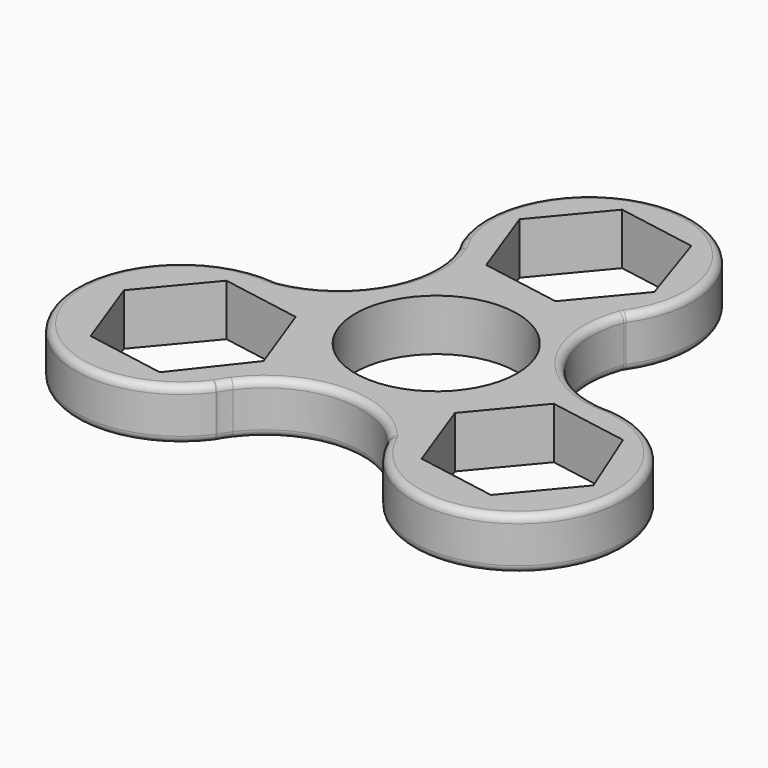
from build123d import *

# Parameters (mm, degrees)
F0_R     = 11
F1_DEPTH = 7
F2_F1_R  = 1
F2_F2_R  = 1
F2_F3_R  = 0.9999


# Not quite as in the source:
# - a fillet or chamfer is up to 0.001 mm smaller than in the source, because OpenCascade refuses the exact size


with BuildPart() as f1:
    # F0 (on Top) → F1 (new body)
    with BuildSketch(Plane.XY):
        with BuildLine():
            ThreePointArc((22.2086241305, 0.0798641866), (12.5198905979, 6.2741646263), (11.4517572715, 17.7240557437))
            ThreePointArc((11.4517572715, 17.7240557437), (1.6771991192, 39.973348249), (-13.0734749912, 20.6603832424))
            ThreePointArc((-13.0734749912, 20.6603832424), (-12.5180191421, 19.6665029377), (-12.0509754633, 18.6281390985))
            ThreePointArc((-12.0509754633, 18.6281390985), (-12.8422160416, 7.2882657582), (-22.2022373142, 0.8377781175))
            ThreePointArc((-22.2022373142, 0.8377781175), (-37.1071375636, -19.0809555006), (-12.384246779, -21.854161524))
            ThreePointArc((-12.384246779, -21.854161524), (-11.9079611923, -21.041379868), (-11.3744869733, -20.2649346104))
            ThreePointArc((-11.3744869733, -20.2649346104), (-1.1159335609, -14.9703009767), (9.3470139898, -19.8485990384))
            ThreePointArc((9.3470139898, -19.8485990384), (34.0495934391, -22.7972544861), (24.0898149129, 0))
            ThreePointArc((24.0898149129, 0), (23.1477825578, 0.0060845895), (22.2086241305, 0.0798641866))
        make_face()
        Polygon((-11.7877372927, -14.5967135669), (-18.7727350589, -23.4860221006), (-29.7069392796, -21.574693228), (-33.5187820314, -11.1497301664), (-26.3964205624, -2.6360959774), (-15.4622163417, -4.5474248499), align=None, mode=Mode.SUBTRACT)
        Polygon((18.388151067, -3.0167495901), (29.3223552878, -4.9280784627), (33.3908597141, -15.0462438958), (26.2684982451, -23.5598780849), (15.3342940244, -21.6485492124), (11.5224512726, -11.2235861508), align=None, mode=Mode.SUBTRACT)
        Circle(F0_R, mode=Mode.SUBTRACT)
        Polygon((-7.122361469, 17.3952310389), (-10.9342042207, 27.8201941005), (-3.8118427518, 36.3338282895), (7.122361469, 34.422499417), (10.6775425462, 23.690738727), (3.8118427518, 15.4839021663), align=None, mode=Mode.SUBTRACT)
    extrude(amount=F1_DEPTH)

    # F2: fillet of radius 1 on 18 edges, made by hand

    # F2_f1
    f2_f1_edges = [f1.edges().sort_by_distance(p)[0] for p in [
        (-22.2022373142, 0.8377781175, 3.5),
        (11.4517572715, 17.7240557437, 3.5),
        (9.3470139898, -19.8485990384, 3.5),
    ]]
    fillet(f2_f1_edges, radius=F2_F1_R)

    # F2_f2
    f2_f2_edges = [f1.edges().sort_by_distance(p)[0] for p in [
        (-13.0734749912, 20.6603832424, 3.5),
        (24.0898149129, 0, 3.5),
        (-12.384246779, -21.854161524, 3.5),
    ]]
    fillet(f2_f2_edges, radius=F2_F2_R)

    # F2_f3 (radius 1 in the source; OpenCascade refuses exactly that, so slightly less here)
    f2_f3_edges = [f1.edges().sort_by_distance(p)[0] for p in [
        (-12.3080271209, 8.3300186134, 7),
        (-12.3080271209, 8.3300186134, 0),
        (1.6570295583, 39.9757483602, 0),
        (1.6570295583, 39.9757483602, 7),
        (13.0595747694, 5.4590227774, 0),
        (13.0595747694, 5.4590227774, 7),
        (34.0685359523, -22.7716924944, 0),
        (34.0685359523, -22.7716924944, 7),
        (-37.094471486, -19.1101411941, 0),
        (-37.094471486, -19.1101411941, 7),
        (-2.0958052267, -15.0267703989, 7),
        (-2.0958052267, -15.0267703989, 0),
        (-12.3875954993, -21.8550114082, 0),
        (9.3360348117, -19.8492368598, 0),
        (9.3360348117, -19.8492368598, 7),
        (-12.3875954993, -21.8550114082, 7),
        (-22.1973000947, 0.8476052754, 7),
        (-22.1973000947, 0.8476052754, 0),
        (24.0922252944, -0.0024751348, 7),
        (24.0922252944, -0.0024751348, 0),
        (11.4571553541, 17.7156429732, 7),
        (11.4571553541, 17.7156429732, 0),
        (-13.0717151079, 20.6647262217, 7),
        (-13.0717151079, 20.6647262217, 0),
    ]]
    fillet(f2_f3_edges, radius=F2_F3_R)


solid = f1.part
